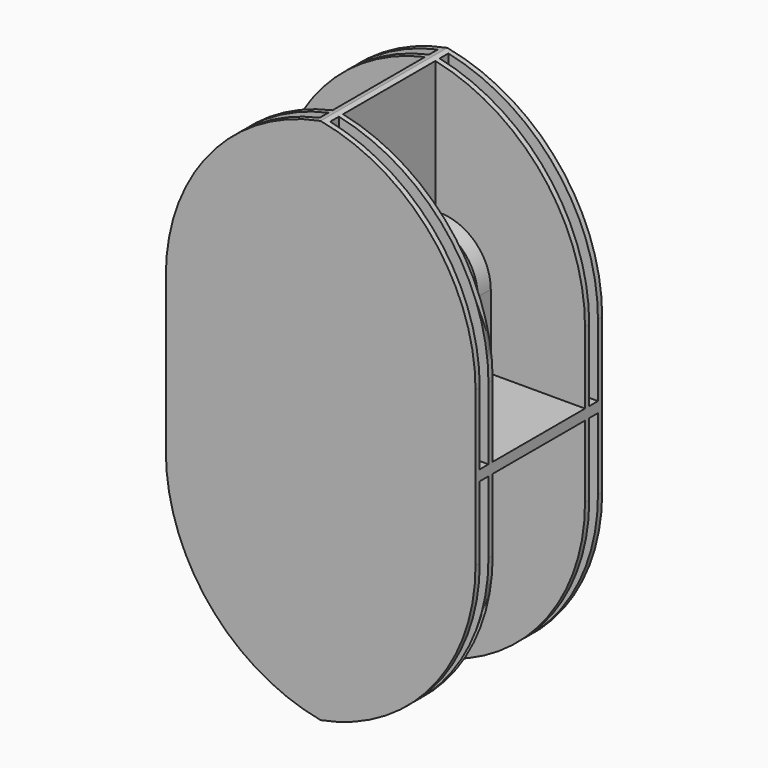
from build123d import *

# Parameters (mm, degrees)
F0_W        = 74.5595730841
F0_H        = 68.4390123934
F1_DEPTH    = 127
F2_T        = -2.54
F3_T1_DEPTH = 451.5844547388
F3_T3_DEPTH = 451.5844547388
F6_W        = 45.6260088831
F6_H        = 7.7898120508
F7_DEPTH    = 76.2
F8_R        = 24.5284097937
F11_W       = 38.0337639379
F11_H       = 74.3822181045
F12_DEPTH   = 5.08


# Not quite as in the source:
# - a fillet or chamfer that OpenCascade refuses, or shapes differently, is made with other operations: its cross-section is extruded or revolved along the edge and cut away or added
# - the program builds the solid bodies; features that only make, move or delete a surface that nothing else refers to are left out


with BuildPart() as f1:
    # F0 (on Top) → F1 (new body)
    with BuildSketch(Plane.XY):
        with Locations((2.225657925, 3.8948999718)):
            Rectangle(F0_W, F0_H)
    extrude(amount=F1_DEPTH)

    # F2
    f2_openings = [f1.faces().sort_by_distance(p)[0] for p in [
        (2.225658, 3.8949, 127),
        (39.505444, 3.8949, 63.5),
    ]]
    offset(amount=F2_T, openings=f2_openings)

    # F3: fillet of radius 91.3683264816 on 2 edges, made by hand

    # F3_s2 → F3_t1 (cut)
    with BuildSketch(Plane.XZ.offset(-196.7376211445)):
        with BuildLine():
            ThreePointArc((-35.054128617, 127), (18.4363311824, 95.5536973082), (39.5054444671, 37.1911090522))
            Line((39.5054444671, 37.1911090522), (39.5054444671, 127))
            Line((39.5054444671, 127), (-35.054128617, 127))
        make_face()
    extrude(amount=F3_T1_DEPTH, mode=Mode.SUBTRACT)

    # F3_s4 → F3_t3 (cut)
    with BuildSketch(Plane.XZ.offset(-262.6366335379)):
        with BuildLine():
            ThreePointArc((-35.054128617, 127), (18.4363311824, 95.5536973082), (39.5054444671, 37.1911090522))
            Line((39.5054444671, 37.1911090522), (39.5054444671, 127))
            Line((39.5054444671, 127), (-35.054128617, 127))
        make_face()
    extrude(amount=F3_T3_DEPTH, mode=Mode.SUBTRACT)

    # F4: F1 across plane


with BuildPart() as f1_1:
    add(f1.part)
    add(f1.part.mirror(Plane.XZ))

    # F5: F1 across plane


with BuildPart() as f1_2:
    add(f1_1.part)
    add(f1_1.part.mirror(Plane.XY))

    # F6 (on face) → F7 (join)
    with BuildSketch(Plane(origin=(0, 0, -2.54), x_dir=(1, 0, 0), z_dir=(0, 0, -1))):
        with Locations((-9.5800887793, 0)):
            Rectangle(F6_W, F6_H)
    extrude(amount=F7_DEPTH)

    # F8
    f8_edges = [f1_2.edges().sort_by_distance(p)[0] for p in [
        (13.232916, 0, -78.74),
    ]]
    fillet(f8_edges, radius=F8_R)

    # F9: F1 across plane


with BuildPart() as f1_3:
    add(f1_2.part)
    add(f1_2.part.mirror(Plane.XY))

    # F10: F1 across face


with BuildPart() as f1_4:
    add(f1_3.part)
    add(f1_3.part.mirror(Plane(origin=(-35.054128617, 0, 0), x_dir=(0, -1, 0), z_dir=(-1, 0, 0))))

    # F11 (on face) → F12 (join)
    with BuildSketch(Plane(origin=(0, 38.1144061685, 0), x_dir=(-1, 0, 0), z_dir=(0, 1, 0))):
        with Locations((32.8460000455, 0)):
            Rectangle(F11_W, F11_H)
    extrude(amount=F12_DEPTH)


solid = f1_4.part
